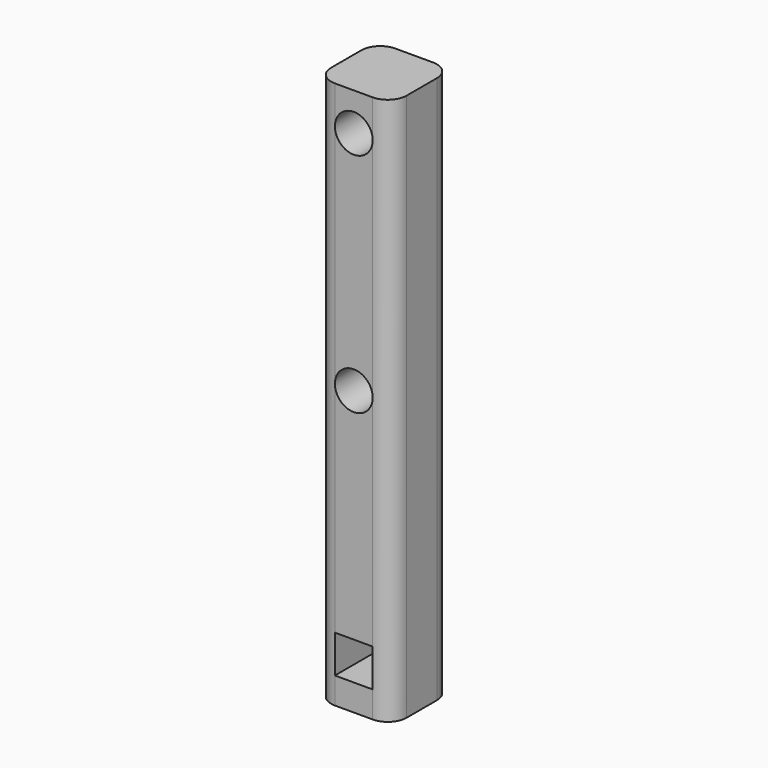
from build123d import *

# Parameters (mm, degrees)
F1_DEPTH = 25.4
F3_D     = 12.7
F3_DEPTH = 254
F3_TIP   = 3.8154649308
F4_W     = 25.4
F4_H     = 82.55
F5_DEPTH = 25.4
F7_DEPTH = 25.4
F8_R     = 6.34999


# Not quite as in the source:
# - a fillet or chamfer is up to 0.001 mm smaller than in the source, because OpenCascade refuses the exact size


with BuildPart() as f1:
    # F0 (on Front) → F1 (new body)
    with BuildSketch(Plane.XZ):
        Polygon((-12.7, -32.0098340811), (0, -32.0098340811), (12.7, -32.0098340811), (12.7, 69.5901659189), (-12.7, 69.5901659189), align=None)
    extrude(amount=F1_DEPTH)

    # F3
    with Locations(Plane.XZ.offset(25.4)):
        with Locations((0, 56.8901659189), (0, -19.3098340811)):
            Hole(F3_D / 2, depth=F3_DEPTH)
            with Locations((0, 0, -(F3_DEPTH + F3_TIP / 2))):  # 118° drill point
                Cone(0, F3_D / 2, F3_TIP, mode=Mode.SUBTRACT)

    # F4 (on face) → F5 (join)
    with BuildSketch(Plane.XZ.offset(25.4)):
        with Locations((0, -73.2848340811)):
            Rectangle(F4_W, F4_H)
    extrude(amount=-F5_DEPTH)

    # F6 (on face) → F7 (cut)
    with BuildSketch(Plane(origin=(0, 0, 0), x_dir=(-1, 0, 0), z_dir=(0, 1, 0))):
        Polygon((0, -105.6698340811), (6.35, -105.6698340811), (6.35, -92.9698340811), (-6.35, -92.9698340811), (-6.35, -105.6698340811), align=None)
    extrude(amount=-F7_DEPTH, mode=Mode.SUBTRACT)

    # F8 (radius 6.35 in the source; OpenCascade refuses exactly that, so slightly less here)
    f8_edges = [f1.edges().sort_by_distance(p)[0] for p in [
        (12.7, 0, -22.484834),
        (-12.7, 0, -22.484834),
        (-12.7, -25.4, -22.484834),
        (12.7, -25.4, -22.484834),
    ]]
    fillet(f8_edges, radius=F8_R)


solid = f1.part
